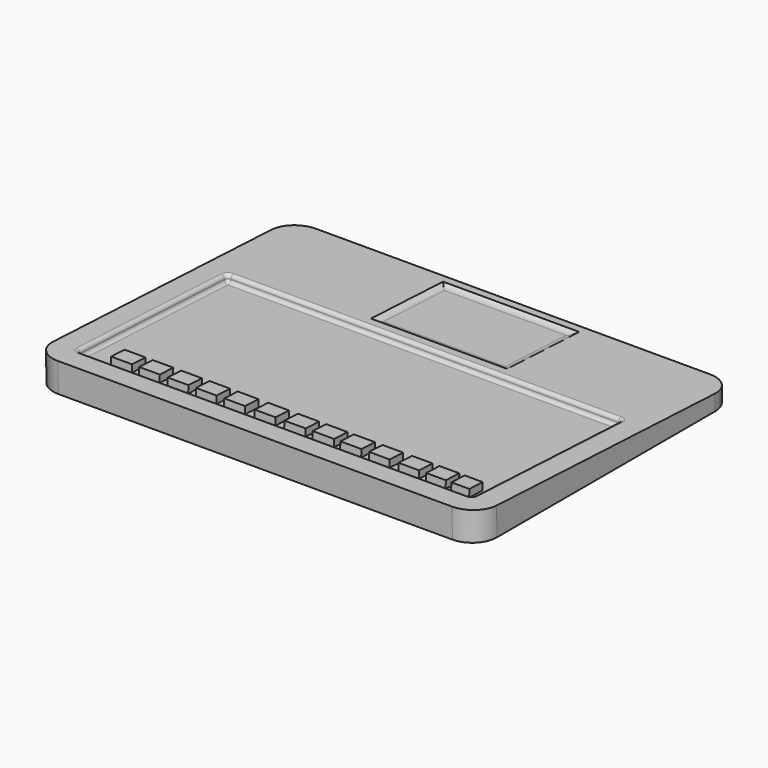
from build123d import *

# Parameters (mm, degrees)
F1_DEPTH     = 30.3
F2_R         = 1.6899494937
F3_W         = 26.949964059
F3_H         = 12.8249995296
F4_DEPTH     = 0.5
F5_R         = 0.2414213562
F6_W         = 1.2325234711
F6_H         = 1.1400654912
F6_W_2       = 1.3488382101
F6_H_2       = 1.1522620916
F6_W_3       = 1.4076605439
F6_W_4       = 1.4072209597
F6_W_5       = 1.4375131577
F6_W_6       = 1.4656018466
F6_W_7       = 1.4457069337
F6_W_8       = 1.4214487746
F6_W_9       = 1.4211460948
F6_W_10      = 1.4119520783
F6_W_11      = 1.4170180075
F6_W_12      = 1.4084377326
F6_W_13      = 1.4295475557
F7_DEPTH     = 0.5
F8_W         = 9.2926481739
F8_H         = 6.1567388475
F9_DEPTH     = 0.19
F10_T1_DEPTH = 11.7376448309
F10_T3_DEPTH = 6.1567388475
F10_T5_DEPTH = 6.1567388475


# Not quite as in the source:
# - a fillet or chamfer that OpenCascade refuses, or shapes differently, is made with other operations: its cross-section is extruded or revolved along the edge and cut away or added


with BuildPart() as f1:
    # F0 (on Right) → F1 (new body)
    with BuildSketch(Plane.YZ):
        Polygon((-44.1633068031, 1.9997905069), (-44.1343598068, 0), (-22.1343598068, 0), (-22.1343598068, 1), align=None)
    extrude(amount=F1_DEPTH)

    # F2
    f2_edges = [f1.edges().sort_by_distance(p)[0] for p in [
        (0, -22.13436, 0.5),
        (30.3, -22.13436, 0.5),
        (30.3, -44.148833, 0.999895),
        (0, -44.148833, 0.999895),
    ]]
    fillet(f2_edges, radius=F2_R)

    # F3 (on face) → F4 (cut)
    with BuildSketch(Plane(origin=(0, -0.0002071974, -0.0045652959), x_dir=(1, 0, 0), z_dir=(0, 0.0453386355, 0.9989716753))):
        with Locations((15.1350684769, -36.10308207)):
            Rectangle(F3_W, F3_H)
    extrude(amount=-F4_DEPTH, mode=Mode.SUBTRACT)

    # F5
    f5_edges = [f1.edges().sort_by_distance(p)[0] for p in [
        (1.660086, -42.483404, 1.67329),
        (28.610051, -42.483404, 1.67329),
        (15.135068, -42.472069, 1.923033),
        (15.135068, -42.494739, 1.423547),
        (1.660086, -36.066164, 1.632299),
        (1.660086, -29.671593, 1.091822),
        (1.660086, -36.088833, 1.132813),
        (28.610051, -29.671593, 1.091822),
        (15.135068, -29.660258, 1.341565),
        (15.135068, -29.682927, 0.842079),
        (28.610051, -36.066164, 1.632299),
        (28.610051, -36.088833, 1.132813),
    ]]
    fillet(f5_edges, radius=F5_R)

    # F6 (on face) → F7 (join)
    with BuildSketch(Plane(origin=(0, -0.0228765151, -0.5040511335), x_dir=(1, 0, 0), z_dir=(0, 0.0453386355, 0.9989716753))):
        with Locations((27.318617329, -41.3098782301)):
            Rectangle(F6_W, F6_H)
        with Locations((25.6510563195, -41.3037799299)):
            Rectangle(F6_W_2, F6_H_2)
        with Locations((23.7977188081, -41.3037799299)):
            Rectangle(F6_W_3, F6_H_2)
        with Locations((21.7823982239, -41.3037799299)):
            Rectangle(F6_W_4, F6_H_2)
        with Locations((19.8403866962, -41.3037799299)):
            Rectangle(F6_W_5, F6_H_2)
        with Locations((17.95785781, -41.3037799299)):
            Rectangle(F6_W_6, F6_H_2)
        with Locations((16.0227976739, -41.3037799299)):
            Rectangle(F6_W_7, F6_H_2)
        with Locations((13.9798414893, -41.3037799299)):
            Rectangle(F6_W_8, F6_H_2)
        with Locations((11.8983006105, -41.3037799299)):
            Rectangle(F6_W_9, F6_H_2)
        with Locations((9.9623361602, -41.3037799299)):
            Rectangle(F6_W_10, F6_H_2)
        with Locations((8.0330308992, -41.3037799299)):
            Rectangle(F6_W_11, F6_H_2)
        with Locations((6.0811268631, -41.3037799299)):
            Rectangle(F6_W_12, F6_H_2)
        with Locations((4.1761151515, -41.3037799299)):
            Rectangle(F6_W_13, F6_H_2)
    extrude(amount=F7_DEPTH)

    # F8 (on face) → F9 (cut)
    with BuildSketch(Plane(origin=(0, -0.0002071974, -0.0045652959), x_dir=(1, 0, 0), z_dir=(0, 0.0453386355, 0.9989716753))):
        with Locations((15.4813206755, -25.8142389357)):
            Rectangle(F8_W, F8_H)
    extrude(amount=-F9_DEPTH, mode=Mode.SUBTRACT)

    # F10: fillet of radius 0.7242640687 on 4 edges, made by hand

    # F10_s2 → F10_t1 (join)
    with BuildSketch(Plane.YZ.offset(9.61249826)):
        with BuildLine():
            ThreePointArc((-28.8631045752, 1.3053861423), (-28.6430306792, 1.1544220499), (-28.3832224346, 1.0934109616))
            Line((-28.3832224346, 1.0934109616), (-28.8717189159, 1.115581524))
            Line((-28.8717189159, 1.115581524), (-28.8631045752, 1.3053861423))
        make_face()
        with BuildLine():
            ThreePointArc((-22.7126968541, 1.026248004), (-22.945540921, 0.8958397321), (-23.2098076761, 0.8586139482))
            Line((-23.2098076761, 0.8586139482), (-22.7213111948, 0.8364433857))
            Line((-22.7213111948, 0.8364433857), (-22.7126968541, 1.026248004))
        make_face()
    extrude(amount=F10_T1_DEPTH)

    # F10_s4 → F10_t3 (join)
    with BuildSketch(Plane(origin=(0, -22.7124896567, 1.0308132999), x_dir=(1, 0, 0), z_dir=(0, -0.9989716753, 0.0453386355))):
        with BuildLine():
            ThreePointArc((10.8349965885, -0.0045699953), (11.061688683, -0.1454009974), (11.3239959199, -0.1945699953))
            Line((11.3239959199, -0.1945699953), (10.8349965885, -0.1945699953))
            Line((10.8349965885, -0.1945699953), (10.8349965885, -0.0045699953))
        make_face()
    extrude(amount=F10_T3_DEPTH)

    # F10_s6 → F10_t5 (join)
    with BuildSketch(Plane(origin=(0, -28.8628973778, 1.3099514382), x_dir=(1, 0, 0), z_dir=(0, 0.9989716753, -0.0453386355))):
        with BuildLine():
            ThreePointArc((20.1276447624, 0.0045699953), (19.9009526679, 0.1454009974), (19.638645431, 0.1945699953))
            Line((19.638645431, 0.1945699953), (20.1276447624, 0.1945699953))
            Line((20.1276447624, 0.1945699953), (20.1276447624, 0.0045699953))
        make_face()
    extrude(amount=F10_T5_DEPTH)


solid = f1.part
